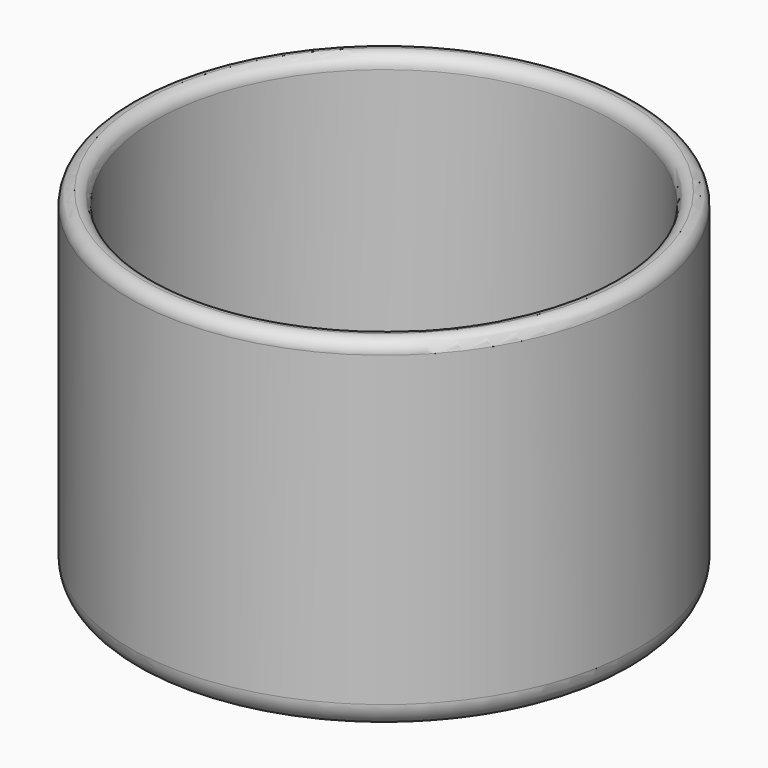
from build123d import *

# Parameters (mm, degrees)
F0_R     = 36.5
F0_W     = 4
F0_H     = 10
F1_DEPTH = 4
F0_R_2   = 40.5
F2_DEPTH = 55
F3_R     = 1.99999
F4_R     = 4


# Not quite as in the source:
# - a fillet or chamfer is up to 0.001 mm smaller than in the source, because OpenCascade refuses the exact size


with BuildPart() as f1:
    # F0 (on Top) → F1 (new body)
    with BuildSketch(Plane.XY):
        Circle(F0_R)
        with Locations((-27.25, -15.4073267064)):
            Rectangle(F0_W, F0_H, mode=Mode.SUBTRACT)
        with Locations((27.25, -14.5926732936)):
            Rectangle(F0_W, F0_H, mode=Mode.SUBTRACT)
        with Locations((-27.25, 14.5926732936)):
            Rectangle(F0_W, F0_H, mode=Mode.SUBTRACT)
        with Locations((27.25, 15.4073267064)):
            Rectangle(F0_W, F0_H, mode=Mode.SUBTRACT)
    extrude(amount=F1_DEPTH)

    # F0 (on Top) → F2 (join)
    with BuildSketch(Plane.XY):
        Circle(F0_R_2)
        Circle(F0_R, mode=Mode.SUBTRACT)
    extrude(amount=F2_DEPTH)

    # F3 (radius 2 in the source; OpenCascade refuses exactly that, so slightly less here)
    f3_edges = [f1.edges().sort_by_distance(p)[0] for p in [
        (-40.5, 0, 55),
        (-36.5, 0, 55),
    ]]
    fillet(f3_edges, radius=F3_R)

    # F4
    f4_edges = [f1.edges().sort_by_distance(p)[0] for p in [
        (-40.5, 0, 0),
    ]]
    fillet(f4_edges, radius=F4_R)


solid = f1.part
